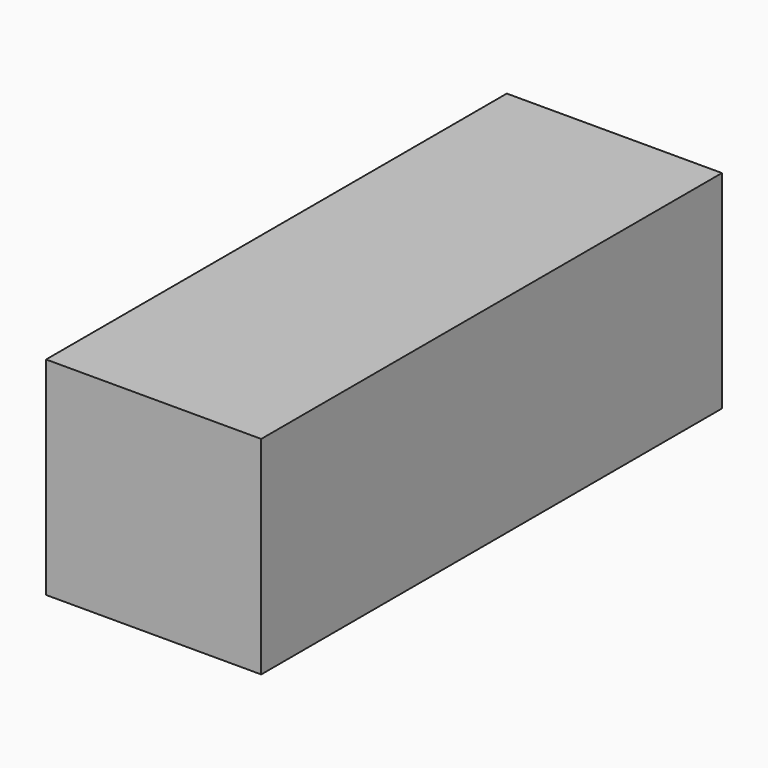
from build123d import *

# Parameters (mm, degrees)
F2_W     = 26.3548903167
F2_H     = 70.5495104194
F3_DEPTH = 25.4


# Not quite as in the source:
# - the program builds the solid bodies; features that only make, move or delete a surface that nothing else refers to are left out


with BuildPart() as f3:
    # F2 (on Top) → F3 (new body)
    with BuildSketch(Plane.XY):
        with Locations((51.7685357481, -0.4414431751)):
            Rectangle(F2_W, F2_H)
    extrude(amount=F3_DEPTH)


solid = f3.part
